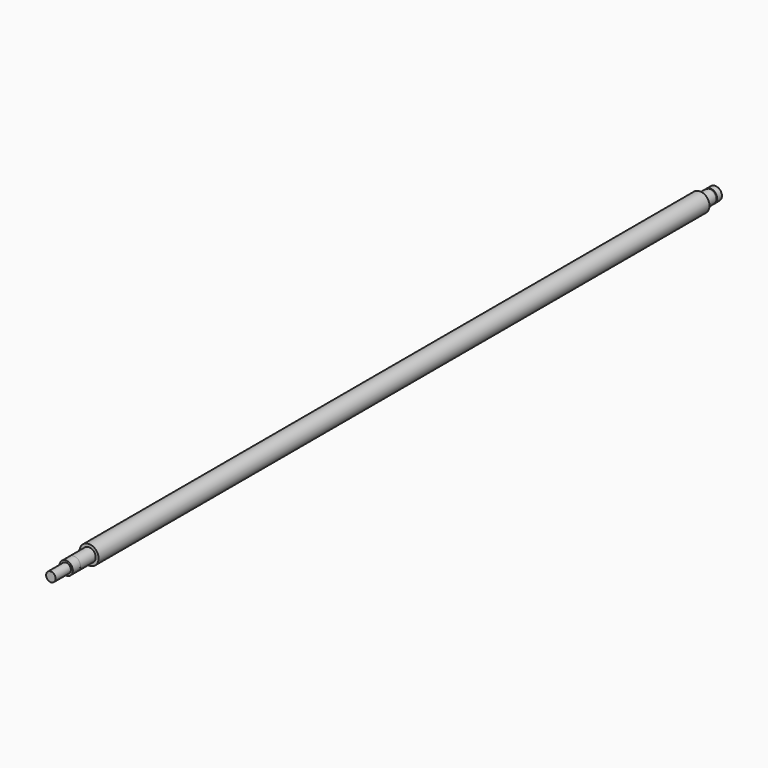
from build123d import *

# Parameters (mm, degrees)
F0_W   = 10
F0_H   = 2.5
F0_W_2 = 0.9
F0_H_2 = 3.25


# Not quite as in the source:
# - a feature names something its author has since deleted; it is built from what else it names


with BuildPart() as f1:
    # F0 (on Right) → F1 (revolve)
    with BuildSketch(Plane.YZ):
        Polygon((200, 3.5), (200, 5), (-200, 5), (-200, 3.5), (-200, 0), (200, 0), align=None)
        Polygon((-200, 0), (-200, 3.5), (-210, 3.5), (-210, 3.48999998), (-210, 0), align=None)
        with Locations((-220, 1.25)):
            Rectangle(F0_W, F0_H)
        Polygon((206, 3.5), (200, 3.5), (200, 0), (206, 0), (206, 3.25), align=None)
        with Locations((206.45, 1.625)):
            Rectangle(F0_W_2, F0_H_2)
        Polygon((206.9, 3.25), (206.9, 0), (210, 0), (210, 3.5), (206.9, 3.5), align=None)
        Polygon((-215, 0), (-210, 0), (-210, 3.48999998), (-215, 3.5), (-215, 2.5), align=None)
    revolve(axis=Axis((0, -7.5, 0), (0, 1, 0)))


solid = f1.part
